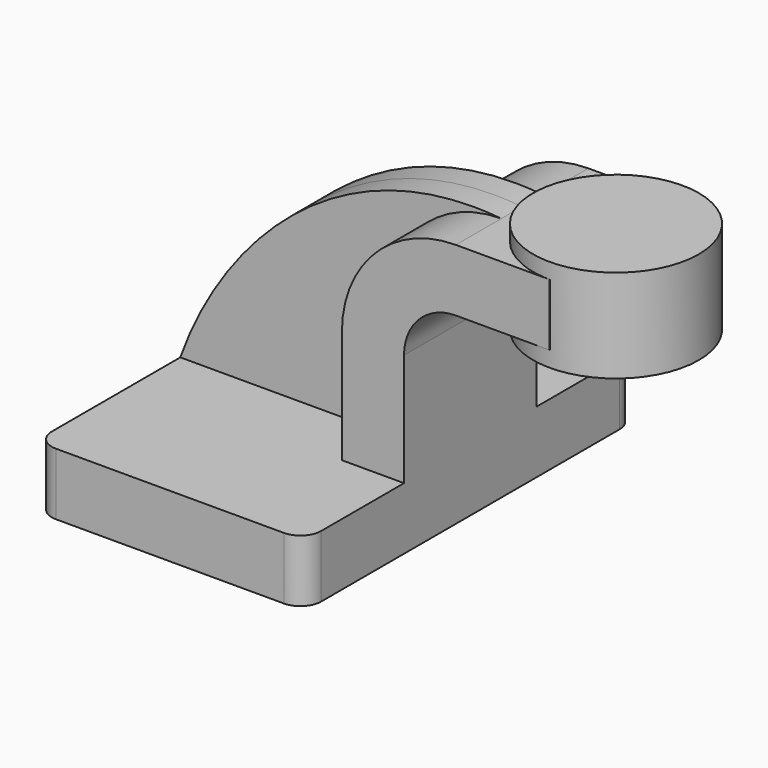
from build123d import *

# Parameters (mm, degrees)
F1_DEPTH = 63.5
F0_W     = 25.4
F0_H     = 19.05
F2_DEPTH = 25.4
F3_DEPTH = 7.9375
F5_R     = 6.35


with BuildPart() as f1:
    # F0 (on Front) → F1 (new body, symmetric)
    with BuildSketch(Plane.XZ):
        Polygon((41.275, -9.525), (41.275, 9.525), (22.225, 9.525), (-41.275, 9.525), (-41.275, -9.525), align=None)
    extrude(amount=F1_DEPTH, both=True)

    # F0 (on Front) → F2 (join, symmetric)
    with BuildSketch(Plane.XZ):
        with BuildLine():
            Line((22.225, 9.525), (41.275, 9.525))
            Line((41.275, 9.525), (41.275, 44.0600354195))
            ThreePointArc((41.275, 44.0600354195), (45.9246798487, 55.2853555708), (57.15, 59.9350354195))
            Line((57.15, 59.9350354195), (60.5272703528, 59.9350354195))
            Line((60.5272703528, 59.9350354195), (60.5272703528, 78.9850354195))
            Line((60.5272703528, 78.9850354195), (57.15, 78.9850354195))
            ThreePointArc((57.15, 78.9850354195), (32.4542956671, 68.7557397524), (22.225, 44.0600354195))
            Line((22.225, 44.0600354195), (22.225, 9.525))
        make_face()
        with Locations((73.2272703528, 69.4600354195)):
            Rectangle(F0_W, F0_H)
    extrude(amount=F2_DEPTH, both=True)

    # F0 (on Front) → F3 (join, symmetric)
    with BuildSketch(Plane.XZ):
        with BuildLine():
            Line((-41.275, 9.525), (22.225, 9.525))
            Line((22.225, 9.525), (22.225, 44.0600354195))
            ThreePointArc((22.225, 44.0600354195), (32.4542956671, 68.7557397524), (57.15, 78.9850354195))
            add(Edge.make_bspline(
                [(-41.275, 9.525), (-28.850948438, 44.7817482054), (6.0363649391, 83.8745053786), (57.15, 78.9850354195)],
                knots=[0, 0, 0, 0, 120.4664980211, 120.4664980211, 120.4664980211, 120.4664980211], degree=3))
        make_face()
    extrude(amount=F3_DEPTH, both=True)

    # F5
    f5_edges = [f1.edges().sort_by_distance(p)[0] for p in [
        (41.275, -63.5, 0),
        (-41.275, -63.5, 0),
        (-41.275, 63.5, 0),
        (41.275, 63.5, 0),
    ]]
    fillet(f5_edges, radius=F5_R)


with BuildPart() as f4:
    # F0 (on Front) → F4 (revolve)
    with BuildSketch(Plane.XZ):
        Polygon((85.9272703528, 78.9850354195), (85.9272703528, 59.9350354195), (85.9272703528, 55.1725354195), (111.3272703528, 55.1725354195), (111.3272703528, 83.7475354195), (85.9272703528, 83.7475354195), align=None)
    revolve(axis=Axis((85.9272703528, 0, 69.4600354195), (0, 0, -1)))


solid = Compound([f1.part, f4.part])
